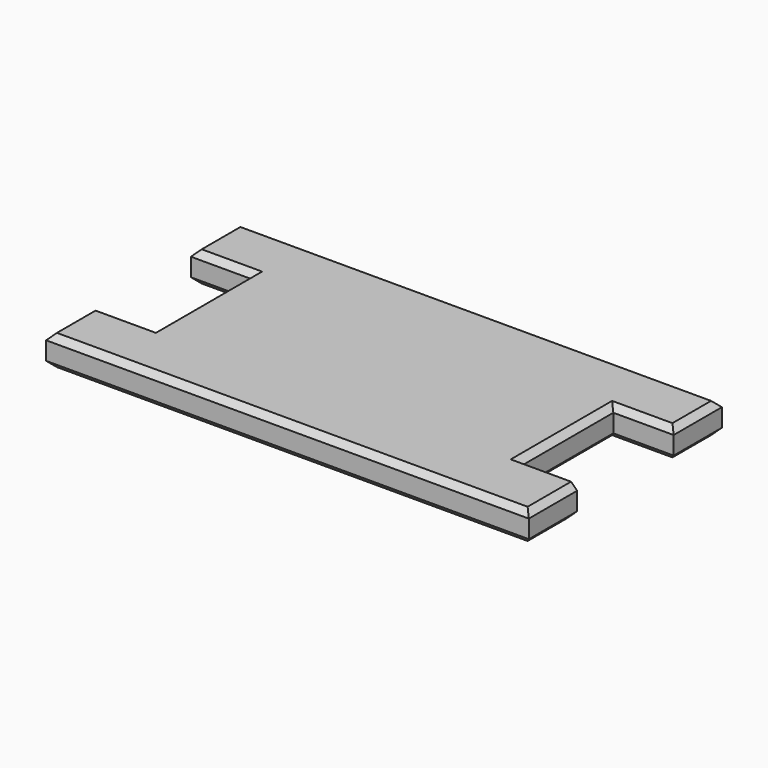
from build123d import *

# Parameters (mm, degrees)
F1_DEPTH = 25
F2_SIZE  = 5
F3_SIZE  = 5
F5_SIZE  = 5


# Not quite as in the source:
# - a feature of the source that left no trace in its solid (it failed there, or was rolled back) is left out


with BuildPart() as f1:
    # F0 (on Top) → F1 (new body)
    with BuildSketch(Plane.XY):
        Polygon((0, 50), (0, 0), (400, 0), (400, 50), (350, 50), (350, 150), (400, 150), (400, 200), (0, 200), (0, 150), (50, 150), (50, 50), align=None)
    extrude(amount=F1_DEPTH)

    # F2
    f2_edges = [f1.edges().sort_by_distance(p)[0] for p in [
        (200, 0, 25),
    ]]
    chamfer(f2_edges, length=F2_SIZE)

    # F3
    f3_edges = [f1.edges().sort_by_distance(p)[0] for p in [
        (200, 200, 25),
    ]]
    chamfer(f3_edges, length=F3_SIZE)

    # F5
    f5_edges = [f1.edges().sort_by_distance(p)[0] for p in [
        (200, 0, 0),
        (200, 200, 0),
        (350, 100, 0),
        (375, 50, 0),
        (400, 25, 0),
        (400, 175, 0),
        (375, 150, 0),
        (0, 175, 0),
        (25, 150, 0),
        (50, 100, 0),
        (25, 50, 0),
        (0, 25, 0),
        (0, 172.5, 25),
        (25, 150, 25),
        (400, 172.5, 25),
        (50, 100, 25),
        (375, 150, 25),
        (25, 50, 25),
        (350, 100, 25),
        (0, 27.5, 25),
        (400, 27.5, 25),
    ]]
    chamfer(f5_edges, length=F5_SIZE)


solid = f1.part
